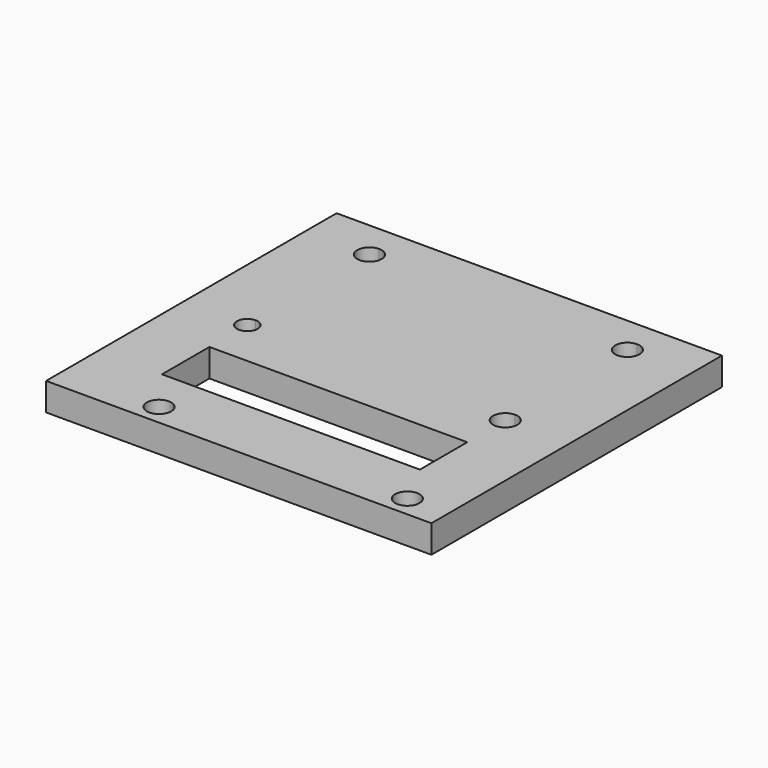
from build123d import *

# Parameters (mm, degrees)
F1_DEPTH = 4.7625


# Not quite as in the source:
# - a length typed as a fraction of an inch, garbled in the dataset ("3 / 203.2 mm" for 3/8 in), is restored


with BuildPart() as f1:
    # F0 (on Top) → F1 (new body)
    with BuildSketch(Plane.XY):
        with BuildLine():
            Line((22.098, 26.5938), (22.098, 31.115))
            Line((22.098, 31.115), (0, 31.115))
            Line((0, 31.115), (-22.098, 31.115))
            Line((-22.098, 31.115), (-22.098, 26.5938))
            ThreePointArc((-22.098, 26.5938), (-20.6252379961, 25.9837620039), (-20.0152, 24.511))
            ThreePointArc((-20.0152, 24.511), (-20.6252379961, 23.0382379961), (-22.098, 22.4282))
            Line((-22.098, 22.4282), (-22.098, 0.127))
            ThreePointArc((-22.098, 0.127), (-20.8407641431, -0.3937641431), (-20.32, -1.651))
            ThreePointArc((-20.32, -1.651), (-20.8407641431, -2.9082358569), (-22.098, -3.429))
            Line((-22.098, -3.429), (-22.098, -9.779))
            Line((-22.098, -9.779), (22.098, -9.779))
            Line((22.098, -9.779), (22.098, -3.7338))
            ThreePointArc((22.098, -3.7338), (20.0152, -1.651), (22.098, 0.4318))
            Line((22.098, 0.4318), (22.098, 22.4282))
            ThreePointArc((22.098, 22.4282), (20.0152, 24.511), (22.098, 26.5938))
        make_face()
        with BuildLine():
            Line((-22.098, 26.5938), (-22.098, 31.115))
            Line((-22.098, 31.115), (-33.02, 31.115))
            Line((-33.02, 31.115), (-33.02, -31.115))
            Line((-33.02, -31.115), (-22.098, -31.115))
            Line((-22.098, -31.115), (-22.098, -27.559))
            Line((-22.098, -27.559), (-22.098, -19.939))
            Line((-22.098, -19.939), (-22.098, -9.779))
            Line((-22.098, -9.779), (-22.098, -3.429))
            ThreePointArc((-22.098, -3.429), (-23.876, -1.651), (-22.098, 0.127))
            Line((-22.098, 0.127), (-22.098, 22.4282))
            ThreePointArc((-22.098, 22.4282), (-24.1808, 24.511), (-22.098, 26.5938))
        make_face()
        with BuildLine():
            Line((33.02, -27.559), (33.02, 31.115))
            Line((33.02, 31.115), (22.098, 31.115))
            Line((22.098, 31.115), (22.098, 26.5938))
            ThreePointArc((22.098, 26.5938), (23.5707620039, 25.9837620039), (24.1808, 24.511))
            ThreePointArc((24.1808, 24.511), (23.5707620039, 23.0382379961), (22.098, 22.4282))
            Line((22.098, 22.4282), (22.098, 0.4318))
            ThreePointArc((22.098, 0.4318), (23.5707620039, -0.1782379961), (24.1808, -1.651))
            ThreePointArc((24.1808, -1.651), (23.5707620039, -3.1237620039), (22.098, -3.7338))
            Line((22.098, -3.7338), (22.098, -9.779))
            Line((22.098, -9.779), (22.098, -19.939))
            Line((22.098, -19.939), (22.098, -27.559))
            Line((22.098, -27.559), (23.9649, -27.559))
            ThreePointArc((23.9649, -27.559), (26.0477, -25.4762), (28.1305, -27.559))
            Line((28.1305, -27.559), (33.02, -27.559))
        make_face()
        with BuildLine():
            Line((33.02, -31.115), (33.02, -27.559))
            Line((33.02, -27.559), (28.1305, -27.559))
            ThreePointArc((28.1305, -27.559), (26.0477, -29.6418), (23.9649, -27.559))
            Line((23.9649, -27.559), (22.098, -27.559))
            Line((22.098, -27.559), (22.098, -31.115))
            Line((22.098, -31.115), (33.02, -31.115))
        make_face()
        with BuildLine():
            Line((-14.4272, -27.559), (22.098, -27.559))
            Line((22.098, -27.559), (22.098, -19.939))
            Line((22.098, -19.939), (-22.098, -19.939))
            Line((-22.098, -19.939), (-22.098, -27.559))
            Line((-22.098, -27.559), (-18.5928, -27.559))
            ThreePointArc((-18.5928, -27.559), (-16.51, -25.4762), (-14.4272, -27.559))
        make_face()
        with BuildLine():
            Line((-22.098, -31.115), (22.098, -31.115))
            Line((22.098, -31.115), (22.098, -27.559))
            Line((22.098, -27.559), (-14.4272, -27.559))
            ThreePointArc((-14.4272, -27.559), (-16.51, -29.6418), (-18.5928, -27.559))
            Line((-18.5928, -27.559), (-22.098, -27.559))
            Line((-22.098, -27.559), (-22.098, -31.115))
        make_face()
    extrude(amount=F1_DEPTH)


solid = f1.part
